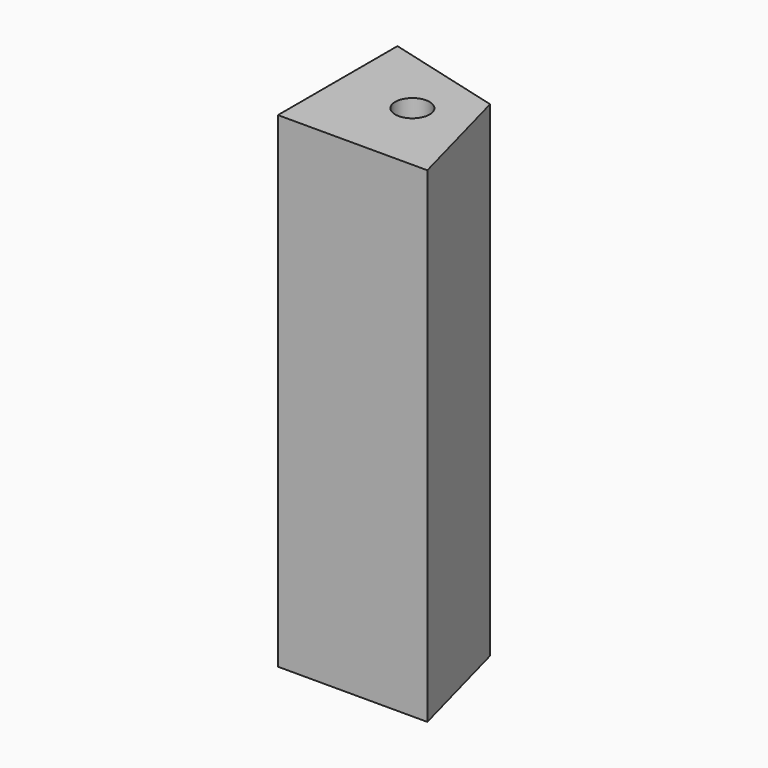
from build123d import *

# Parameters (mm, degrees)
F0_R     = 1.4605
F1_DEPTH = 20.6375


# Not quite as in the source:
# - a length typed as a fraction of an inch, garbled in the dataset ("3 / 203.2 mm" for 3/8 in), is restored


with BuildPart() as f1:
    # F0 (on Top) → F1 (new body, symmetric)
    with BuildSketch(Plane.XY):
        Polygon((-6.35, -6.35), (6.35, -6.35), (3.6661742094, 3.6661742094), (-6.35, 6.35), align=None)
        Circle(F0_R, mode=Mode.SUBTRACT)
    extrude(amount=F1_DEPTH, both=True)


solid = f1.part
